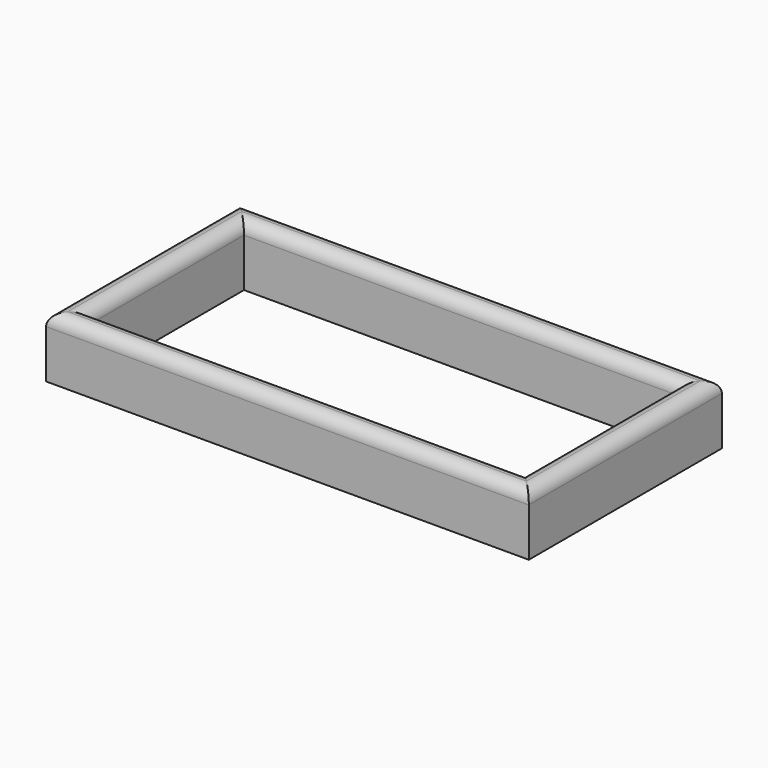
from build123d import *

# Parameters (mm, degrees)
F0_W     = 200
F0_H     = 100
F0_W_2   = 180
F0_H_2   = 80
F1_DEPTH = 25
F2_R     = 4.99999


# Not quite as in the source:
# - a fillet or chamfer is up to 0.001 mm smaller than in the source, because OpenCascade refuses the exact size


with BuildPart() as f1:
    # F0 (on Top) → F1 (new body)
    with BuildSketch(Plane.XY):
        Rectangle(F0_W, F0_H)
        Rectangle(F0_W_2, F0_H_2, mode=Mode.SUBTRACT)
    extrude(amount=F1_DEPTH)

    # F2 (radius 5 in the source; OpenCascade refuses exactly that, so slightly less here)
    f2_edges = [f1.edges().sort_by_distance(p)[0] for p in [
        (-100, 0, 25),
        (0, 50, 25),
        (0, -50, 25),
        (100, 0, 25),
        (90, 0, 25),
        (0, -40, 25),
        (-90, 0, 25),
        (0, 40, 25),
    ]]
    fillet(f2_edges, radius=F2_R)


solid = f1.part
